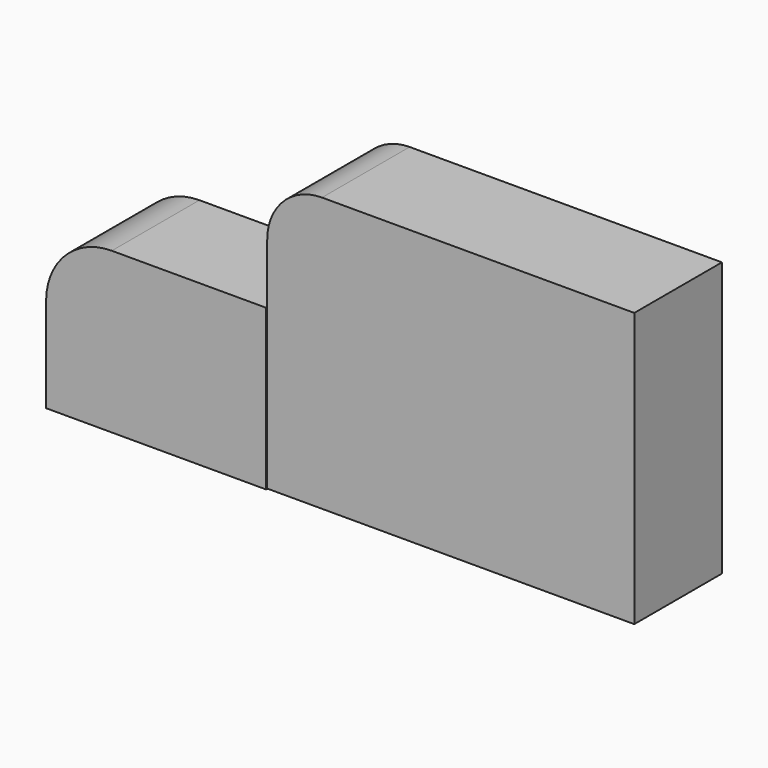
from build123d import *

# Parameters (mm, degrees)
F2_DEPTH = 25.4
F3_DEPTH = 25.4
F7_W     = 37.0916780084
F7_H     = 3.1564831734
F7_W_2   = 56.6421654075
F8_DEPTH = 2.54


# Not quite as in the source:
# - the program builds the solid bodies; features that only make, move or delete a surface that nothing else refers to are left out


with BuildPart() as f2:
    # F0 (on Front) → F2 (new body)
    with BuildSketch(Plane.XZ):
        with BuildLine():
            Line((65.2430579066, 24.3388270795), (-7.1682546616, 24.3388270795))
            ThreePointArc((-7.1682546616, 24.3388270795), (-16.1485107826, 20.6190832006), (-19.8682546616, 11.6388270795))
            Line((-19.8682546616, 11.6388270795), (-19.8682546616, -39.1995310783))
            Line((-19.8682546616, -39.1995310783), (65.2430579066, -39.1995310783))
            Line((65.2430579066, -39.1995310783), (65.2430579066, 24.3388270795))
        make_face()
    extrude(amount=F2_DEPTH)


with BuildPart() as f3:
    # F1 (on Front) → F3 (new body)
    with BuildSketch(Plane.XZ):
        with BuildLine():
            Line((-20.1367456466, -39.4680202007), (-20.1367456466, -2.3737917019))
            Line((-20.1367456466, -2.3737917019), (-55.9098335004, -2.3737917019))
            ThreePointArc((-55.9098335004, -2.3737917019), (-66.6861408457, -6.8374843567), (-71.1498335004, -17.6137917019))
            Line((-71.1498335004, -17.6137917019), (-71.1498335004, -39.4680202007))
            Line((-71.1498335004, -39.4680202007), (-20.1367456466, -39.4680202007))
        make_face()
    extrude(amount=F3_DEPTH)

    # F7 (on face) → F8 (join)
    with BuildSketch(Plane(origin=(0, 0, -39.4680202007), x_dir=(1, 0, 0), z_dir=(0, 0, -1))):
        with Locations((-38.6825846508, 13.3175728843)):
            Rectangle(F7_W, F7_H)
        with Locations((8.1843370572, 13.3175728843)):
            Rectangle(F7_W_2, F7_H)
    extrude(amount=F8_DEPTH)


solid = Compound([f2.part, f3.part])
